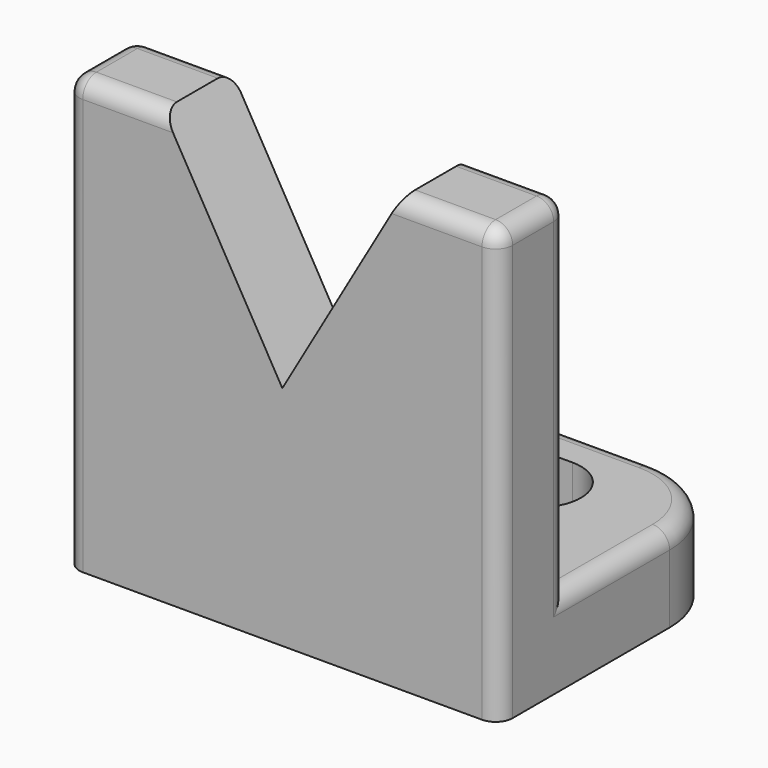
from build123d import *

# Parameters (mm, degrees)
F1_DEPTH = 2.5
F3_DEPTH = 5
F4_R     = 1


# Not quite as in the source:
# - a feature names something its author has since deleted; it is built from what else it names


with BuildPart() as f1:
    # F0 (on Front) → F1 (new body, symmetric)
    with BuildSketch(Plane.XZ):
        Polygon((-6.985, -1.9016251091), (-12.7, -1.9016251091), (-12.7, -27.3016251091), (12.7, -27.3016251091), (12.7, -1.9016251091), (6.985, -1.9016251091), (0, -14), align=None)
    extrude(amount=F1_DEPTH, both=True)

    # F2 (on face) → F3 (join)
    with BuildSketch(Plane(origin=(0, 0, -27.3016251091), x_dir=(1, 0, 0), z_dir=(0, 0, -1))):
        with BuildLine():
            ThreePointArc((-12.7, -10), (-11.2355339059, -13.5355339059), (-7.7, -15))
            Line((-7.7, -15), (7.7, -15))
            ThreePointArc((7.7, -15), (11.2355339059, -13.5355339059), (12.7, -10))
            Line((12.7, -10), (12.7, -2.5))
            Line((12.7, -2.5), (-12.7, -2.5))
            Line((-12.7, -2.5), (-12.7, -10))
        make_face()
        with BuildLine():
            Line((-5, -7.5), (5, -7.5))
            ThreePointArc((5, -7.5), (7.5, -10), (5, -12.5))
            Line((5, -12.5), (-5, -12.5))
            ThreePointArc((-5, -12.5), (-7.5, -10), (-5, -7.5))
        make_face(mode=Mode.SUBTRACT)
    extrude(amount=-F3_DEPTH)

    # F4
    f4_edges = [f1.edges().sort_by_distance(p)[0] for p in [
        (-12.7, -2.5, -14.601625),
        (-9.8425, -2.5, -1.901625),
        (-12.7, 0, -1.901625),
        (-9.8425, 2.5, -1.901625),
        (-12.7, 2.5, -12.101625),
        (-12.7, 6.25, -22.301625),
        (12.7, 2.5, -12.101625),
        (12.7, -2.5, -14.601625),
        (12.7, 0, -1.901625),
        (9.8425, 2.5, -1.901625),
        (9.8425, -2.5, -1.901625),
    ]]
    fillet(f4_edges, radius=F4_R)


solid = f1.part
